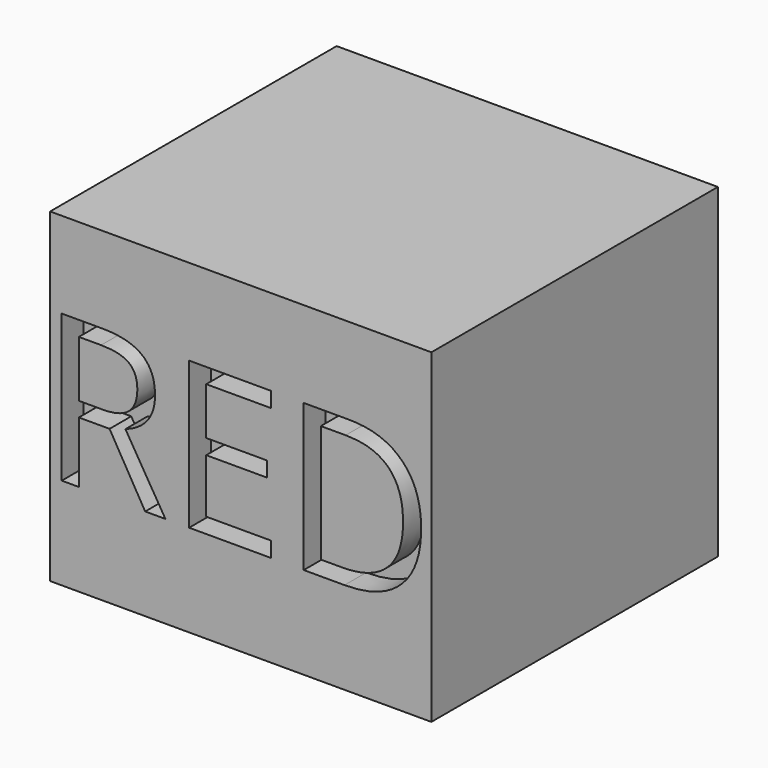
from build123d import *

# Parameters (mm, degrees)
F0_W         = 89.2803221941
F0_H         = 83.8607475162
F1_DEPTH     = 76.2
F2_TEXT_SIZE = 48.2578456319
F3_DEPTH     = 6.35


# Not quite as in the source:
# - Text() gives the source's letters only with a copy of the font that has no kerning and outlines rounded to 1/6400 em; it was checked with that copy


with BuildPart() as f1:
    # F0 (on Top) → F1 (new body)
    with BuildSketch(Plane.XY):
        with Locations((0.1426190138, -0.7131025195)):
            Rectangle(F0_W, F0_H)
    extrude(amount=F1_DEPTH)

    # F2 (on face) → F3 (cut)
    with BuildSketch(Plane.XZ.offset(42.6434762776)):
        with Locations((-46.5101902136, 21.588292429)):
            Text('RED', F2_TEXT_SIZE, font='Open Sans', text_align=(TextAlign.LEFT, TextAlign.BOTTOM))
    extrude(amount=-F3_DEPTH, mode=Mode.SUBTRACT)


solid = f1.part
